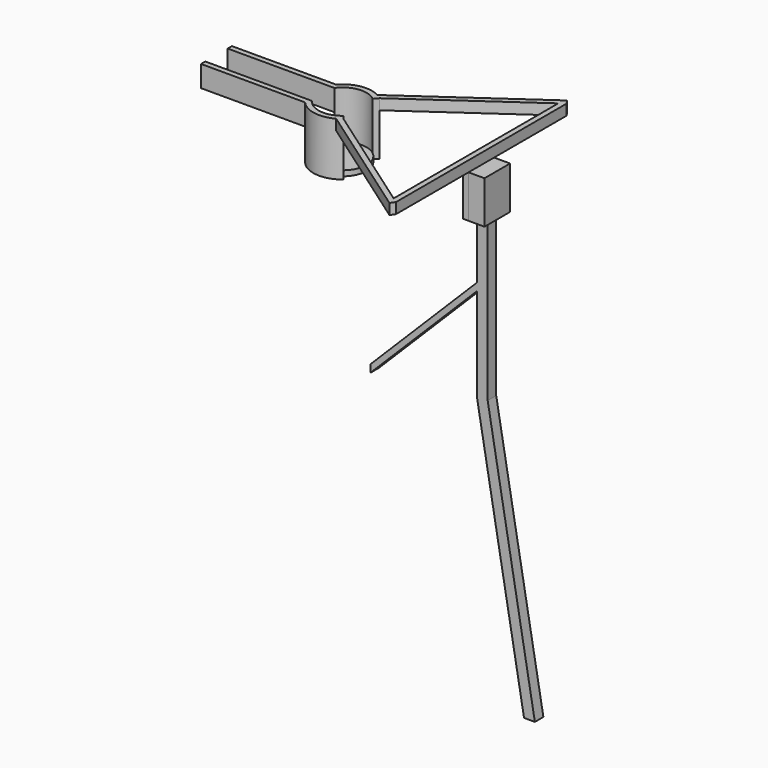
from build123d import *

# Parameters (mm, degrees)
F1_DEPTH  = 2
F2_DEPTH  = 4
F3_DEPTH  = 10
F5_R      = 4.5
F6_DEPTH  = 1
F7_W      = 6
F7_H      = 8
F7_R      = 1.3
F8_DEPTH  = 1
F9_DEPTH  = 3
F10_DEPTH = 1.5
F12_DEPTH = 1


with BuildPart() as f1:
    # F0 (on Top) → F1 (new body)
    with BuildSketch(Plane.XY):
        Polygon((-23.6550478793, -2.625), (-23.6550478793, -3.625), (-4.1363480269, -3.625), (-3.6550478793, -2.625), align=None)
        with BuildLine():
            Line((-3.6550478793, -2.625), (-4.1363480269, -3.625))
            ThreePointArc((-4.1363480269, -3.625), (-0.9506837802, -5.4172133381), (2.6548679611, -4.81681182))
            ThreePointArc((2.6548679611, -4.81681182), (3.1097776177, -4.5364394814), (3.5353318533, -4.2132444372))
            Line((3.5353318533, -4.2132444372), (2.8925442436, -3.447199994))
            ThreePointArc((2.8925442436, -3.447199994), (-0.5606747329, -4.4649349204), (-3.6550478793, -2.625))
        make_face()
        with BuildLine():
            ThreePointArc((3.5353318533, -4.2132444372), (3.1097776177, -4.5364394814), (2.6548679611, -4.81681182))
            Line((2.6548679611, -4.81681182), (25.4251697083, -20.8127749449))
            Line((25.4251697083, -20.8127749449), (26, -19.9945022912))
            Line((26, -19.9945022912), (25, -19.9945022912))
            Line((25, -19.9945022912), (25, -19.2920099262))
            Line((25, -19.2920099262), (3.5353318533, -4.2132444372))
        make_face()
        Polygon((25, 0), (25, -19.2920099262), (26, -19.9945022912), (26, 0), align=None)
        Polygon((26, -19.9945022912), (25, -19.2920099262), (25, -19.9945022912), align=None)
    extrude(amount=-F1_DEPTH)

    # F0 (on Top) → F2 (join)
    with BuildSketch(Plane.XY):
        Polygon((-23.6550478793, -2.625), (-23.6550478793, -3.625), (-4.1363480269, -3.625), (-3.6550478793, -2.625), align=None)
        with BuildLine():
            Line((-3.6550478793, -2.625), (-4.1363480269, -3.625))
            ThreePointArc((-4.1363480269, -3.625), (-0.9506837802, -5.4172133381), (2.6548679611, -4.81681182))
            ThreePointArc((2.6548679611, -4.81681182), (3.1097776177, -4.5364394814), (3.5353318533, -4.2132444372))
            Line((3.5353318533, -4.2132444372), (2.8925442436, -3.447199994))
            ThreePointArc((2.8925442436, -3.447199994), (-0.5606747329, -4.4649349204), (-3.6550478793, -2.625))
        make_face()
    extrude(amount=-F2_DEPTH)

    # F0 (on Top) → F3 (join)
    with BuildSketch(Plane.XY):
        with BuildLine():
            Line((-3.6550478793, -2.625), (-4.1363480269, -3.625))
            ThreePointArc((-4.1363480269, -3.625), (-0.9506837802, -5.4172133381), (2.6548679611, -4.81681182))
            ThreePointArc((2.6548679611, -4.81681182), (3.1097776177, -4.5364394814), (3.5353318533, -4.2132444372))
            Line((3.5353318533, -4.2132444372), (2.8925442436, -3.447199994))
            ThreePointArc((2.8925442436, -3.447199994), (-0.5606747329, -4.4649349204), (-3.6550478793, -2.625))
        make_face()
    extrude(amount=-F3_DEPTH)

    # F4: F1 across plane


with BuildPart() as f1_1:
    add(f1.part)
    add(f1.part.mirror(Plane.XZ))

    # F5 (on face) → F6 (join)
    with BuildSketch(Plane(origin=(0, 0, -10), x_dir=(1, 0, 0), z_dir=(0, 0, -1))):
        Circle(F5_R)
    extrude(amount=-F6_DEPTH)

    # F7 (on face) → F8 (join, through all)
    with BuildSketch(Plane.YZ.offset(26)):
        with Locations((0, -6)):
            Rectangle(F7_W, F7_H)
        with Locations((0, -8)):
            Circle(F7_R, mode=Mode.SUBTRACT)
        with Locations((0, -4)):
            Circle(F7_R, mode=Mode.SUBTRACT)
    extrude(amount=-F8_DEPTH)


with BuildPart() as f9:
    # F7 (on face) → F9 (new body)
    with BuildSketch(Plane.YZ.offset(26)):
        with Locations((0, -6)):
            Rectangle(F7_W, F7_H)
        with Locations((0, -8)):
            Circle(F7_R, mode=Mode.SUBTRACT)
        with Locations((0, -4)):
            Circle(F7_R, mode=Mode.SUBTRACT)
        with Locations((0, -4)):
            Circle(F7_R)
        with Locations((0, -8)):
            Circle(F7_R)
    extrude(amount=F9_DEPTH)

    # F7 (on face) → F10 (join)
    with BuildSketch(Plane.YZ.offset(26)):
        with Locations((0, -4)):
            Circle(F7_R)
        with Locations((0, -8)):
            Circle(F7_R)
    extrude(amount=-F10_DEPTH)

    # F11 (on Front) → F12 (join, symmetric)
    with BuildSketch(Plane.XZ):
        Polygon((28, -10), (26, -10), (26, -21), (6, -41), (6, -42.4142135624), (26, -22.4142135624), (26, -40), (34.8163490354, -90), (36.8472022592, -90), (28, -39.8250226729), align=None)
    extrude(amount=F12_DEPTH, both=True)


solid = Compound([f1_1.part, f9.part])
